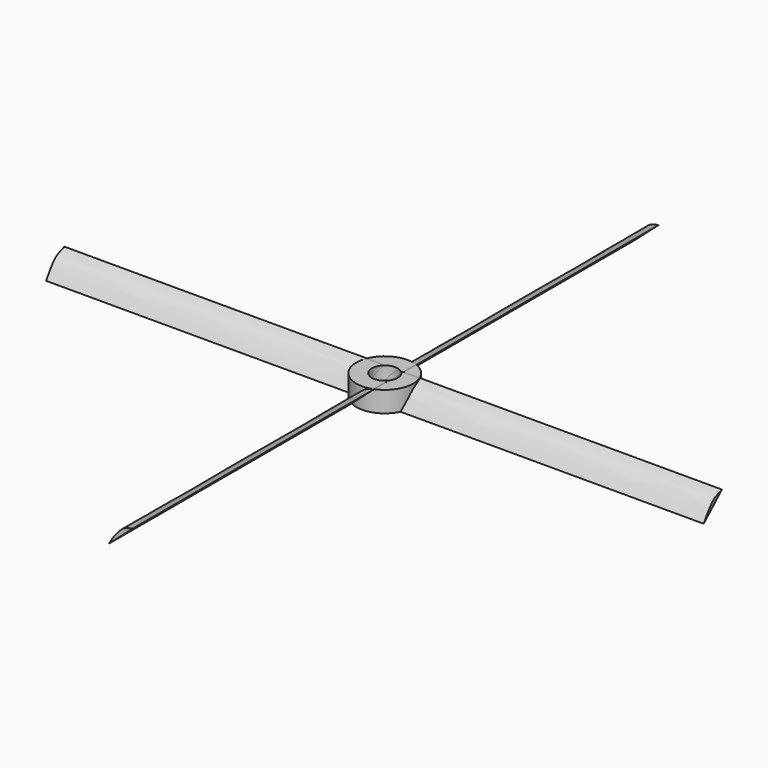
from build123d import *
from build123d import SkipClean  # not in build123d's __all__

# Parameters (mm, degrees)
F0_R     = 5.5
F0_R_2   = 2.5
F1_DEPTH = 4
F4_DEPTH = 63.5
F5_DEPTH = 63.5
F6_DEPTH = 25.4


with BuildPart() as f1:
    # F0 (on Top) → F1 (new body)
    with BuildSketch(Plane.XY):
        Circle(F0_R)
        Circle(F0_R_2, mode=Mode.SUBTRACT)
    extrude(amount=F1_DEPTH)

    # F2 (on Right) → F4 (join, symmetric)
    with BuildSketch(Plane.YZ):
        with BuildLine():
            add(Edge.make_bspline(
                [(2.0092245694, 4.03282993), (1.2332558193, 3.6627267699), (-0.1709254175, 3.5531850395), (-1.7467354882, 1.0394306207), (-2.3899459585, 0)],
                knots=[0, 0, 0, 0, 0.4279448525, 1, 1, 1, 1], degree=3))
            Line((-2.3899459585, 0), (2.0092245694, 4.03282993))
        make_face()
    extrude(amount=F4_DEPTH, both=True)

    # F3 (on Front) → F5 (join, symmetric)
    with BuildSketch(Plane.XZ):
        with BuildLine():
            add(Edge.make_bspline(
                [(2.0786884706, 4.0288106538), (1.3651493792, 3.9074184187), (0.0363126012, 3.7460034701), (-1.7134352279, 1.3773564618), (-2.4795364588, 0)],
                knots=[0, 0, 0, 0, 0.3998148531, 1, 1, 1, 1], degree=3))
            Line((-2.4795364588, 0), (2.0786884706, 4.0288106538))
        make_face()
    extrude(amount=F5_DEPTH, both=True)

    # F0 (on Top) → F6 (cut)
    with BuildSketch(Plane.XY):
        Circle(F0_R_2)
    with SkipClean():  # cleaning this boolean's faces spoils the solid; the shape is the same uncleaned
        extrude(amount=F6_DEPTH, mode=Mode.SUBTRACT)


solid = f1.part
